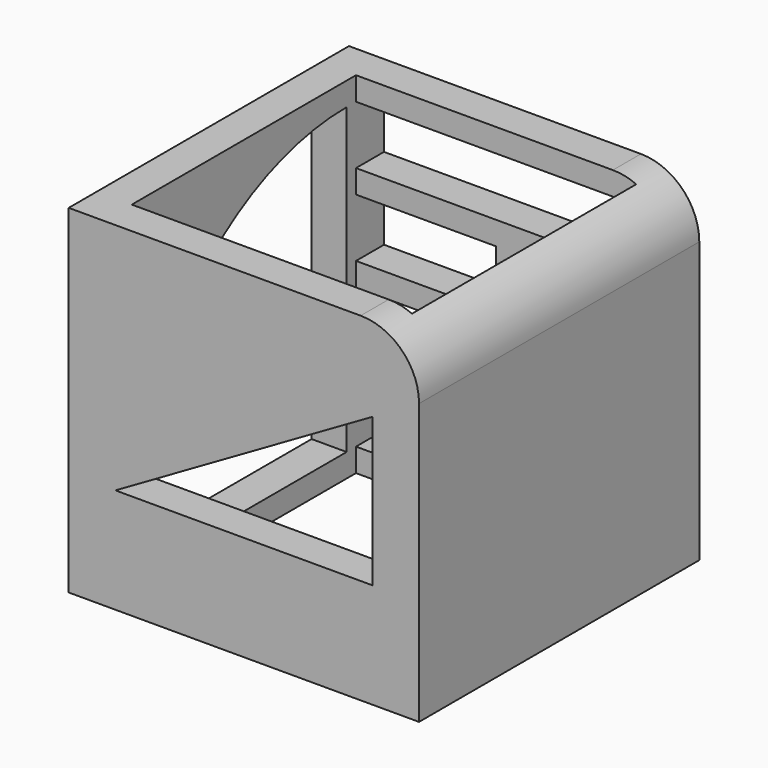
from build123d import *

# Parameters (mm, degrees)
F0_W          = 30
F0_H          = 30
F0_W_2        = 24
F0_H_2        = 24
F1_DEPTH      = 30
F3_DEPTH      = 5
F5_DEPTH      = 4
F6_W          = 12
F6_H          = 5
F6_W_2        = 6
F6_W_3        = 3
F6_W_4        = 24
F7_DEPTH      = 3
F8_W          = 30.8
F8_H          = 30.8
F8_W_2        = 27
F8_H_2        = 27
F9_DEPTH      = 1
F10_T1_DEPTH  = 27
F10_T3_DEPTH  = 27
F10_T9_DEPTH  = 30.7080992435
F10_T14_DEPTH = 30.7080992435
F10_T22_DEPTH = 30.7080992435
F10_T27_DEPTH = 30.7080992435
F10_T35_DEPTH = 30.7080992435
F10_T40_DEPTH = 30.7080992435
F10_T48_DEPTH = 30.7080992435
F10_T53_DEPTH = 30.7080992435
F11_T1_DEPTH  = 55


# Not quite as in the source:
# - a fillet or chamfer that OpenCascade refuses, or shapes differently, is made with other operations: its cross-section is extruded or revolved along the edge and cut away or added


with BuildPart() as f1:
    # F0 (on Top) → F1 (new body)
    with BuildSketch(Plane.XY):
        Rectangle(F0_W, F0_H)
        Rectangle(F0_W_2, F0_H_2, mode=Mode.SUBTRACT)
    extrude(amount=F1_DEPTH)

    # F2 (on face) → F3 (cut)
    with BuildSketch(Plane.XZ.offset(15)):
        Polygon((11, 22.7017059222), (-11, 10), (11, 10), align=None)
    extrude(amount=-F3_DEPTH, mode=Mode.SUBTRACT)

    # F4 (on face) → F5 (cut)
    with BuildSketch(Plane(origin=(-15, 0, 0), x_dir=(0, -1, 0), z_dir=(-1, 0, 0))):
        with BuildLine():
            ThreePointArc((11, 2), (6.0293863659, 20.1017884635), (-11, 28))
            Line((-11, 28), (-11, 2))
            Line((-11, 2), (11, 2))
        make_face()
    extrude(amount=-F5_DEPTH, mode=Mode.SUBTRACT)

    # F6 (on face) → F7 (cut)
    with BuildSketch(Plane(origin=(0, 15, 0), x_dir=(-1, 0, 0), z_dir=(0, 1, 0))):
        with Locations((6, 18.5)):
            Rectangle(F6_W, F6_H)
        with Locations((9, 11.5)):
            Rectangle(F6_W_2, F6_H)
        with Locations((10.5, 4.5)):
            Rectangle(F6_W_3, F6_H)
        with Locations((0, 25.5)):
            Rectangle(F6_W_4, F6_H)
    extrude(amount=-F7_DEPTH, mode=Mode.SUBTRACT)

    # F8 (on face) → F9 (cut)
    with BuildSketch(Plane(origin=(0, 0, 0), x_dir=(1, 0, 0), z_dir=(0, 0, -1))):
        Rectangle(F8_W, F8_H)
        Rectangle(F8_W_2, F8_H_2, mode=Mode.SUBTRACT)
    extrude(amount=-F9_DEPTH, mode=Mode.SUBTRACT)

    # F10: fillet of radius 1.6 on 4 edges, made by hand

    # F10_s2 → F10_t1 (join)
    with BuildSketch(Plane.XZ.offset(-13.5)):
        with BuildLine():
            ThreePointArc((-14.9832396974, 1), (-14.0888125064, 0.7266499161), (-13.5, 0))
            Line((-13.5, 0), (-13.5, 1))
            Line((-13.5, 1), (-14.9832396974, 1))
        make_face()
        with BuildLine():
            ThreePointArc((14.9832396974, 1), (14.0888125064, 0.7266499161), (13.5, 0))
            Line((13.5, 0), (13.5, 1))
            Line((13.5, 1), (14.9832396974, 1))
        make_face()
    extrude(amount=F10_T1_DEPTH)

    # F10_s4 → F10_t3 (join)
    with BuildSketch(Plane.YZ.offset(-13.5)):
        with BuildLine():
            ThreePointArc((14.9832396974, 1), (14.0888125064, 0.7266499161), (13.5, 0))
            Line((13.5, 0), (13.5, 1))
            Line((13.5, 1), (14.9832396974, 1))
        make_face()
        with BuildLine():
            ThreePointArc((-14.9832396974, 1), (-14.0888125064, 0.7266499161), (-13.5, 0))
            Line((-13.5, 0), (-13.5, 1))
            Line((-13.5, 1), (-14.9832396974, 1))
        make_face()
    extrude(amount=F10_T3_DEPTH)


with BuildPart() as f10_tool7:
    # F10_s8 → F10_t9 (new body)
    with BuildSketch(Plane.XZ.offset(-17.2080992435)):
        with BuildLine():
            ThreePointArc((-14.9832396974, 1), (-14.0888125064, 0.7266499161), (-13.5, 0))
            Line((-13.5, 0), (-13.5, 1))
            Line((-13.5, 1), (-14.9832396974, 1))
        make_face()
    extrude(amount=F10_T9_DEPTH)

    split(bisect_by=Plane.XZ.offset(-15), keep=Keep.TOP)

    split(bisect_by=Plane.XZ.offset(-13.5), keep=Keep.BOTTOM)


with BuildPart() as f10_tool12:
    # F10_s13 → F10_t14 (new body)
    with BuildSketch(Plane.YZ.offset(13.5)):
        with BuildLine():
            ThreePointArc((14.9832396974, 1), (14.0888125064, 0.7266499161), (13.5, 0))
            Line((13.5, 0), (13.5, 1))
            Line((13.5, 1), (14.9832396974, 1))
        make_face()
    extrude(amount=-F10_T14_DEPTH)

    split(bisect_by=Plane.YZ.offset(-15), keep=Keep.TOP)

    split(bisect_by=Plane.YZ.offset(-13.5), keep=Keep.BOTTOM)


with BuildPart() as f10_tool7_1:
    add(f10_tool7.part)

    # F10_t17: intersect F10_tool12
    add(f10_tool12.part, mode=Mode.INTERSECT)


with BuildPart() as f1_1:
    add(f1.part)

    # F10_t5: union F10_tool7
    add(f10_tool7_1.part)


with BuildPart() as f10_tool20:
    # F10_s21 → F10_t22 (new body)
    with BuildSketch(Plane.XZ.offset(-13.5)):
        with BuildLine():
            ThreePointArc((-14.9832396974, 1), (-14.0888125064, 0.7266499161), (-13.5, 0))
            Line((-13.5, 0), (-13.5, 1))
            Line((-13.5, 1), (-14.9832396974, 1))
        make_face()
    extrude(amount=F10_T22_DEPTH)

    split(bisect_by=Plane.XZ.offset(15), keep=Keep.BOTTOM)

    split(bisect_by=Plane.XZ.offset(13.5), keep=Keep.TOP)


with BuildPart() as f10_tool25:
    # F10_s26 → F10_t27 (new body)
    with BuildSketch(Plane.YZ.offset(-17.2080992435)):
        with BuildLine():
            ThreePointArc((-14.9832396974, 1), (-14.0888125064, 0.7266499161), (-13.5, 0))
            Line((-13.5, 0), (-13.5, 1))
            Line((-13.5, 1), (-14.9832396974, 1))
        make_face()
    extrude(amount=F10_T27_DEPTH)

    split(bisect_by=Plane.YZ.offset(-15), keep=Keep.TOP)

    split(bisect_by=Plane.YZ.offset(-13.5), keep=Keep.BOTTOM)


with BuildPart() as f10_tool20_1:
    add(f10_tool20.part)

    # F10_t30: intersect F10_tool25
    add(f10_tool25.part, mode=Mode.INTERSECT)


with BuildPart() as f1_2:
    add(f1_1.part)

    # F10_t18: union F10_tool20
    add(f10_tool20_1.part)


with BuildPart() as f10_tool33:
    # F10_s34 → F10_t35 (new body)
    with BuildSketch(Plane.YZ.offset(17.2080992435)):
        with BuildLine():
            ThreePointArc((14.9832396974, 1), (14.0888125064, 0.7266499161), (13.5, 0))
            Line((13.5, 0), (13.5, 1))
            Line((13.5, 1), (14.9832396974, 1))
        make_face()
    extrude(amount=-F10_T35_DEPTH)

    split(bisect_by=Plane.YZ.offset(15), keep=Keep.BOTTOM)

    split(bisect_by=Plane.YZ.offset(13.5), keep=Keep.TOP)


with BuildPart() as f10_tool38:
    # F10_s39 → F10_t40 (new body)
    with BuildSketch(Plane.XZ.offset(13.5)):
        with BuildLine():
            ThreePointArc((14.9832396974, 1), (14.0888125064, 0.7266499161), (13.5, 0))
            Line((13.5, 0), (13.5, 1))
            Line((13.5, 1), (14.9832396974, 1))
        make_face()
    extrude(amount=-F10_T40_DEPTH)

    split(bisect_by=Plane.XZ.offset(-15), keep=Keep.TOP)

    split(bisect_by=Plane.XZ.offset(-13.5), keep=Keep.BOTTOM)


with BuildPart() as f10_tool33_1:
    add(f10_tool33.part)

    # F10_t43: intersect F10_tool38
    add(f10_tool38.part, mode=Mode.INTERSECT)


with BuildPart() as f1_3:
    add(f1_2.part)

    # F10_t31: union F10_tool33
    add(f10_tool33_1.part)


with BuildPart() as f10_tool46:
    # F10_s47 → F10_t48 (new body)
    with BuildSketch(Plane.YZ.offset(-13.5)):
        with BuildLine():
            ThreePointArc((-14.9832396974, 1), (-14.0888125064, 0.7266499161), (-13.5, 0))
            Line((-13.5, 0), (-13.5, 1))
            Line((-13.5, 1), (-14.9832396974, 1))
        make_face()
    extrude(amount=F10_T48_DEPTH)

    split(bisect_by=Plane.YZ.offset(15), keep=Keep.BOTTOM)

    split(bisect_by=Plane.YZ.offset(13.5), keep=Keep.TOP)


with BuildPart() as f10_tool51:
    # F10_s52 → F10_t53 (new body)
    with BuildSketch(Plane.XZ.offset(17.2080992435)):
        with BuildLine():
            ThreePointArc((14.9832396974, 1), (14.0888125064, 0.7266499161), (13.5, 0))
            Line((13.5, 0), (13.5, 1))
            Line((13.5, 1), (14.9832396974, 1))
        make_face()
    extrude(amount=-F10_T53_DEPTH)

    split(bisect_by=Plane.XZ.offset(15), keep=Keep.BOTTOM)

    split(bisect_by=Plane.XZ.offset(13.5), keep=Keep.TOP)


with BuildPart() as f10_tool46_1:
    add(f10_tool46.part)

    # F10_t56: intersect F10_tool51
    add(f10_tool51.part, mode=Mode.INTERSECT)


with BuildPart() as f1_4:
    add(f1_3.part)

    # F10_t44: union F10_tool46
    add(f10_tool46_1.part)

    # F11: fillet of radius 5 on 1 edges, made by hand

    # F11_s2 → F11_t1 (cut)
    with BuildSketch(Plane.XZ.offset(-27.5)):
        with BuildLine():
            ThreePointArc((15, 25), (13.5355339059, 28.5355339059), (10, 30))
            Line((10, 30), (15, 30))
            Line((15, 30), (15, 25))
        make_face()
    extrude(amount=F11_T1_DEPTH, mode=Mode.SUBTRACT)


solid = f1_4.part
